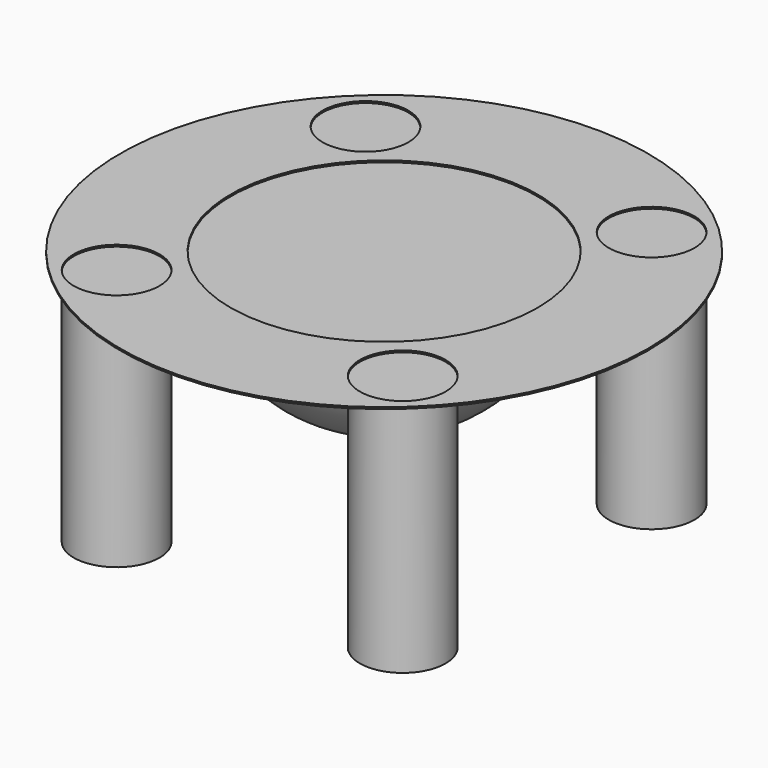
from build123d import *

# Parameters (mm, degrees)
F0_R     = 1.23825
F1_DEPTH = 6.858
F0_R_2   = 4.4323
F2_DEPTH = 4.1148
F0_R_3   = 7.62
F4_DEPTH = 0.0508


# Not quite as in the source:
# - a fillet or chamfer that OpenCascade refuses, or shapes differently, is made with other operations: its cross-section is extruded or revolved along the edge and cut away or added


with BuildPart() as f1:
    # F0 (on Top) → F1 (new body)
    with BuildSketch(Plane.XY):
        with Locations((-4.1298802341, 4.4900714386)):
            Circle(F0_R)
    extrude(amount=-F1_DEPTH)


with BuildPart() as f1b:
    # F0 (on Top) → F1, piece 2 (new body)
    with BuildSketch(Plane.XY):
        with Locations((-4.1298802341, -4.4900714386)):
            Circle(F0_R)
    extrude(amount=-F1_DEPTH)


with BuildPart() as f1c:
    # F0 (on Top) → F1, piece 3 (new body)
    with BuildSketch(Plane.XY):
        with Locations((4.1298802341, -4.4900714386)):
            Circle(F0_R)
    extrude(amount=-F1_DEPTH)


with BuildPart() as f1d:
    # F0 (on Top) → F1, piece 4 (new body)
    with BuildSketch(Plane.XY):
        with Locations((4.1298802341, 4.4900714386)):
            Circle(F0_R)
    extrude(amount=-F1_DEPTH)


with BuildPart() as f2:
    # F0 (on Top) → F2 (new body)
    with BuildSketch(Plane.XY):
        Circle(F0_R_2)
    extrude(amount=-F2_DEPTH)

    # F3: fillet of radius 4.4151137629 on 1 edges, made by hand

    # F3_s1 → F3_t2 (revolve, cut)
    with BuildSketch(Plane.XZ):
        with BuildLine():
            ThreePointArc((4.4323, 0), (3.041321932, -2.9260734556), (0.0274116719, -4.1148))
            Line((0.0274116719, -4.1148), (4.4323, -4.1148))
            Line((4.4323, -4.1148), (4.4323, 0))
        make_face()
    revolve(axis=Axis((0, 0, -4.1148), (0, 0, 1)), mode=Mode.SUBTRACT)


with BuildPart() as f4:
    # F0 (on Top) → F4 (new body)
    with BuildSketch(Plane.XY):
        Circle(F0_R_3)
        with Locations((-4.1298802341, -4.4900714386)):
            Circle(F0_R, mode=Mode.SUBTRACT)
        with Locations((4.1298802341, -4.4900714386)):
            Circle(F0_R, mode=Mode.SUBTRACT)
        with Locations((-4.1298802341, 4.4900714386)):
            Circle(F0_R, mode=Mode.SUBTRACT)
        Circle(F0_R_2, mode=Mode.SUBTRACT)
        with Locations((4.1298802341, 4.4900714386)):
            Circle(F0_R, mode=Mode.SUBTRACT)
    extrude(amount=F4_DEPTH)


solid = Compound([f1.part, f1b.part, f1c.part, f1d.part, f2.part, f4.part])
